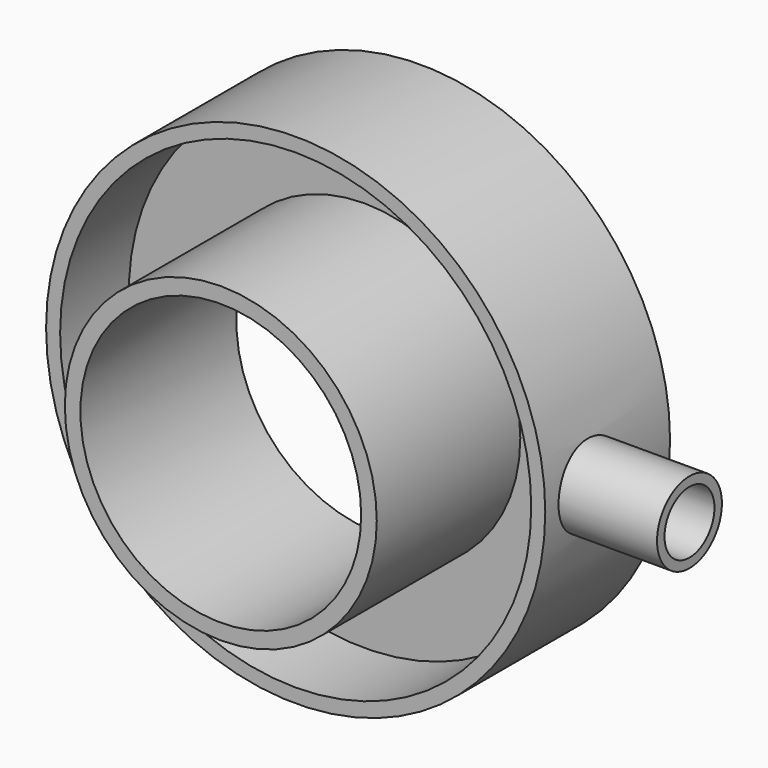
from build123d import *

# Parameters (mm, degrees)
F0_R      = 40
F0_R_2    = 37.75
F1_DEPTH  = 15
F2_DEPTH  = 10
F0_R_3    = 25
F3_DEPTH  = 1.25
F0_R_4    = 22.5
F4_DEPTH  = 30
F5_DEPTH  = 1.25
F7_R      = 5
F8_DEPTH  = 39
F9_R      = 5
F11_R     = 6.5
F11_R_2   = 5
F12_DEPTH = 17
F13_DEPTH = 10


with BuildPart() as f1:
    # F0 (on Front) → F1 (new body)
    with BuildSketch(Plane.XZ):
        with Locations((-137.480571866, 0)):
            Circle(F0_R)
        with Locations((-137.480571866, 0)):
            Circle(F0_R_2, mode=Mode.SUBTRACT)
    extrude(amount=F1_DEPTH)

    # F2 (add): a face of the model
    f2_faces = [f1.faces().sort_by_distance(p)[0] for p in [
        (-176.3492010161, 0, 0),
    ]]
    extrude(f2_faces, amount=F2_DEPTH)

    # F0 (on Front) → F3 (join, symmetric)
    with BuildSketch(Plane.XZ):
        with Locations((-137.480571866, 0)):
            Circle(F0_R_2)
        with Locations((-137.480571866, 0)):
            Circle(F0_R_3, mode=Mode.SUBTRACT)
    extrude(amount=F3_DEPTH, both=True)

    # F0 (on Front) → F4 (join)
    with BuildSketch(Plane.XZ):
        with Locations((-137.480571866, 0)):
            Circle(F0_R_3)
        with Locations((-137.480571866, 0)):
            Circle(F0_R_4, mode=Mode.SUBTRACT)
    extrude(amount=F4_DEPTH)

    # F5 (add): a face of the model
    f5_faces = [f1.faces().sort_by_distance(p)[0] for p in [
        (-161.7734650848, 0, 0),
    ]]
    extrude(f5_faces, amount=F5_DEPTH)

    # F7 (on offset) → F8 (cut)
    with BuildSketch(Plane.YZ.offset(-107.4)):
        with Locations((-5.8384072036, 0)):
            Circle(F7_R)
    extrude(amount=F8_DEPTH, mode=Mode.SUBTRACT)

    # F9
    f9_edges = [f1.edges().sort_by_distance(p)[0] for p in [
        (-103.59144, -1.25, 1.986585),
        (-103.59144, -1.25, -1.986585),
    ]]
    fillet(f9_edges, radius=F9_R)

    # F11 (on offset) → F12 (join)
    with BuildSketch(Plane.YZ.offset(-98.7)):
        with Locations((-5.8384072036, 0)):
            Circle(F11_R)
        with Locations((-5.8384072036, 0)):
            Circle(F11_R_2, mode=Mode.SUBTRACT)
    extrude(amount=F12_DEPTH)

    # F11 (on offset) → F13 (join)
    with BuildSketch(Plane.YZ.offset(-98.7)):
        with Locations((-5.8384072036, 0)):
            Circle(F11_R)
        with Locations((-5.8384072036, 0)):
            Circle(F11_R_2, mode=Mode.SUBTRACT)
    extrude(amount=F13_DEPTH)


solid = f1.part
